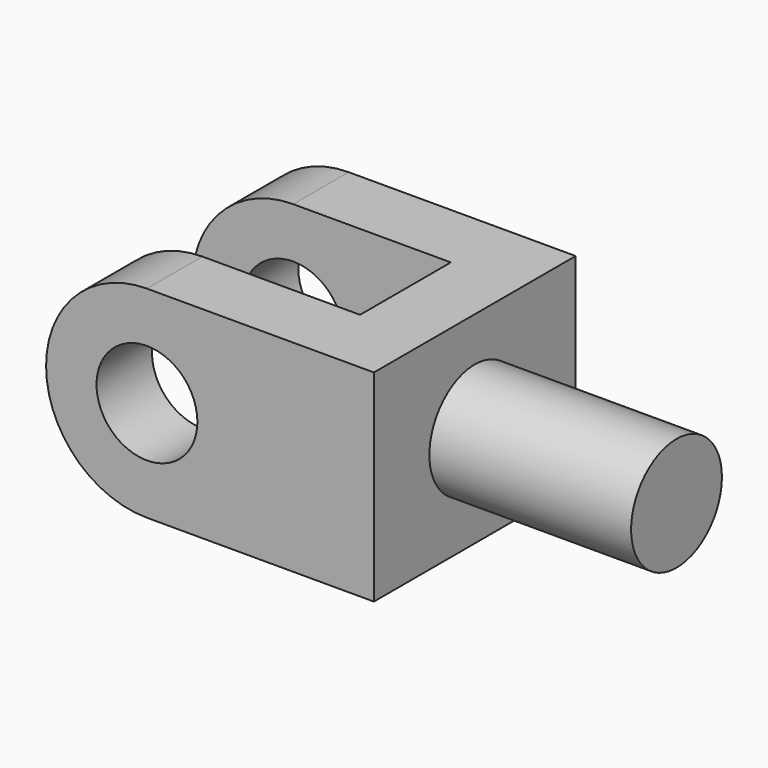
from build123d import *

# Parameters (mm, degrees)
F0_R      = 228.6
F1_DEPTH  = 812.8
F3_DEPTH  = 406.4
F4_DEPTH  = 406.4
F6_DEPTH  = 279.4
F8_DEPTH  = 279.4
F9_R      = 203.2
F10_DEPTH = 279.4
F11_R     = 203.2
F12_DEPTH = 279.4


# Not quite as in the source:
# - a pattern or mirror of a feature is missing from the dataset's text; its kind, count and spacing are read off the source's solid


with BuildPart() as f1:
    # F0 (on Right) → F1 (new body)
    with BuildSketch(Plane.YZ):
        Circle(F0_R)
    extrude(amount=F1_DEPTH)

    # F2 (on Top) → F3 (join)
    with BuildSketch(Plane.XY):
        Polygon((0, -508), (0, 0), (0, 508), (-914.4, 508), (-914.4, 228.6), (-279.4, 228.6), (-279.4, -228.6), (-914.4, -228.6), (-914.4, -508), align=None)
    extrude(amount=F3_DEPTH)

    # F4 (add): a face of the model
    f4_faces = [f1.faces().sort_by_distance(p)[0] for p in [
        (-13.6688820318, 368.3, 0),
    ]]
    extrude(f4_faces, amount=F4_DEPTH)

    # F5 (on face) → F6 (join)
    with BuildSketch(Plane.XZ.offset(508)):
        with BuildLine():
            Line((-914.4, -406.4), (-914.4, 406.4))
            ThreePointArc((-914.4, 406.4), (-1320.8, 0), (-914.4, -406.4))
        make_face()
    f6 = extrude(amount=-F6_DEPTH)

    # F6_copies: F6 across plane
    add(f6.mirror(Plane.ZX))

    # F7 (on face) → F8 (join)
    with BuildSketch(Plane(origin=(0, 508, 0), x_dir=(-1, 0, 0), z_dir=(0, 1, 0))):
        with BuildLine():
            ThreePointArc((914.4, -406.4), (1201.7681958742, -287.3681958742), (1320.8, 0))
            ThreePointArc((1320.8, 0), (1201.7681958742, 287.3681958742), (914.4, 406.4))
            Line((914.4, 406.4), (914.4, -406.4))
        make_face()
    extrude(amount=-F8_DEPTH)

    # F9 (on face) → F10 (cut)
    with BuildSketch(Plane.XZ.offset(508)):
        with Locations((-914.4, 0)):
            Circle(F9_R)
    extrude(amount=-F10_DEPTH, mode=Mode.SUBTRACT)

    # F11 (on face) → F12 (cut)
    with BuildSketch(Plane(origin=(0, 508, 0), x_dir=(-1, 0, 0), z_dir=(0, 1, 0))):
        with Locations((914.4, 0)):
            Circle(F11_R)
    extrude(amount=-F12_DEPTH, mode=Mode.SUBTRACT)


solid = f1.part
